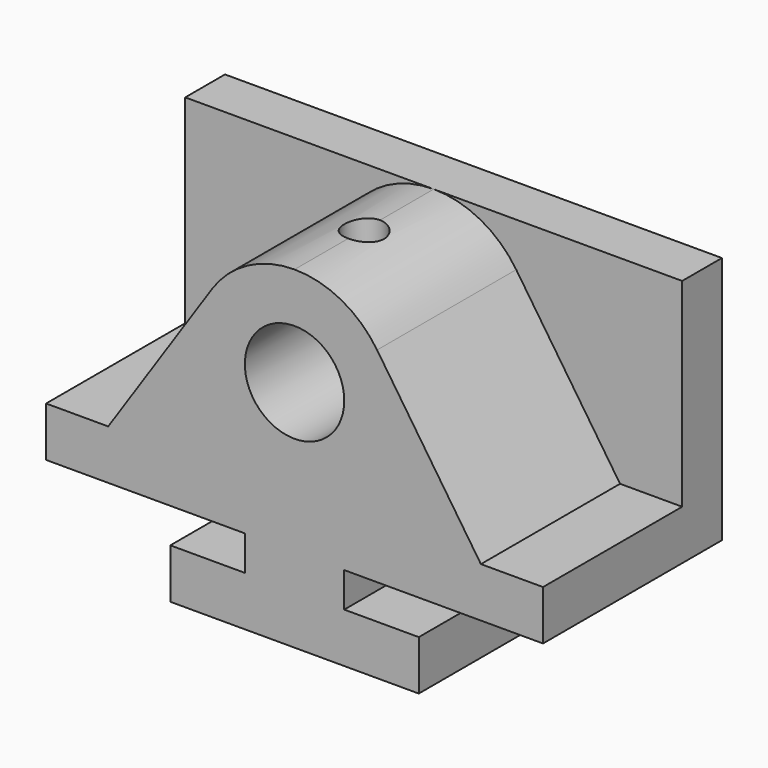
from build123d import *
from build123d import SkipClean  # not in build123d's __all__

# Parameters (mm, degrees)
F0_W     = 127
F0_H     = 85.09
F1_DEPTH = 57.15
F3_DEPTH = 57.151
F4_R     = 12.7
F5_DEPTH = 44.45
F6_R     = 5.08
F7_REACH = 99.4594097937


with BuildPart() as f1:
    # F0 (on Front) → F1 (new body)
    with BuildSketch(Plane.XZ):
        with Locations((63.5, 42.545)):
            Rectangle(F0_W, F0_H)
    extrude(amount=F1_DEPTH)

    # F2 (on face) → F3 (cut, through all)
    with BuildSketch(Plane.XZ.offset(57.15)):
        Polygon((0, 0), (31.75, 0), (31.75, 12.7), (50.8, 12.7), (50.8, 21.59), (0, 21.59), align=None)
        Polygon((95.25, 12.7), (95.25, 0), (127, 0), (127, 21.59), (76.2, 21.59), (76.2, 12.7), align=None)
    extrude(amount=-F3_DEPTH, mode=Mode.SUBTRACT)

    # F4 (on face) → F5 (cut)
    with BuildSketch(Plane.XZ.offset(57.15)):
        with Locations((63.5, 59.69)):
            Circle(F4_R)
        with BuildLine():
            Line((0, 85.09), (0, 34.29))
            Line((0, 34.29), (15.875, 34.29))
            Line((15.875, 34.29), (42.4065743945, 73.8401730104))
            ThreePointArc((42.4065743945, 73.8401730104), (51.5470588235, 82.1017647059), (63.5, 85.09))
            Line((63.5, 85.09), (0, 85.09))
        make_face()
        with BuildLine():
            Line((127, 85.09), (63.5, 85.09))
            ThreePointArc((63.5, 85.09), (75.4529411765, 82.1017647059), (84.5934256055, 73.8401730104))
            Line((84.5934256055, 73.8401730104), (111.125, 34.29))
            Line((111.125, 34.29), (127, 34.29))
            Line((127, 34.29), (127, 85.09))
        make_face()
    extrude(amount=-F5_DEPTH, mode=Mode.SUBTRACT)

    f7_end = f1.faces().sort_by_distance((50.8, -34.925, 59.69))[0]
    # F6 (on face) → F7 (cut, up to a face of the model that its end follows)
    with BuildSketch(Plane.XY.offset(85.09)):
        with Locations((63.5, -34.925)):
            Circle(F6_R)
    f7_long = extrude(amount=-F7_REACH, mode=Mode.PRIVATE)
    add(split(f7_long, bisect_by=f7_end, keep=Keep.ALL, mode=Mode.PRIVATE).solids().sort_by_distance((63.5, -34.925, 85.09))[0], mode=Mode.SUBTRACT)


solid = f1.part
